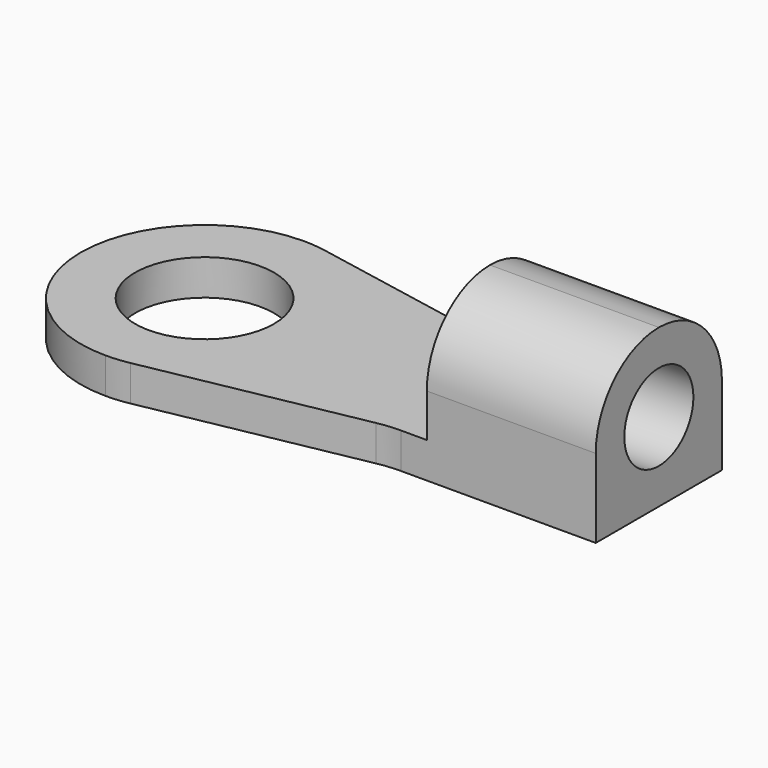
from build123d import *

# Parameters (mm, degrees)
F0_R     = 1.85
F1_DEPTH = 0.95
F2_W     = 4.5
F2_H     = 4.2
F3_DEPTH = 3.25
F4_R     = 2.09999
F5_R     = 1.15
F6_DEPTH = 25


# Not quite as in the source:
# - a fillet or chamfer is up to 0.001 mm smaller than in the source, because OpenCascade refuses the exact size


with BuildPart() as f1:
    # F0 (on Top) → F1 (new body)
    with BuildSketch(Plane.XY):
        with BuildLine():
            Line((10.9, 1.2), (15.4, 1.2))
            Line((15.4, 1.2), (15.4, 5.4))
            Line((15.4, 5.4), (10.9, 5.4))
            Line((10.9, 5.4), (10.2120730928, 5.4))
            ThreePointArc((10.2120730928, 5.4), (9.9013861494, 5.4146577616), (9.5934591909, 5.4585008344))
            Line((9.5934591909, 5.4585008344), (3.9186139019, 6.5414991656))
            ThreePointArc((3.9186139019, 6.5414991656), (3.6106869434, 6.5853422384), (3.3, 6.6))
            ThreePointArc((3.3, 6.6), (0.9665476221, 5.6334523779), (0, 3.3))
            ThreePointArc((0, 3.3), (0.9665476221, 0.9665476221), (3.3, 0))
            ThreePointArc((3.3, 0), (3.6106869434, 0.0146577616), (3.9186139019, 0.0585008344))
            Line((3.9186139019, 0.0585008344), (9.5934591909, 1.1414991656))
            ThreePointArc((9.5934591909, 1.1414991656), (9.9013861494, 1.1853422384), (10.2120730928, 1.2))
            Line((10.2120730928, 1.2), (10.9, 1.2))
        make_face()
        with Locations((3.3, 3.3)):
            Circle(F0_R, mode=Mode.SUBTRACT)
    extrude(amount=F1_DEPTH)

    # F2 (on face) → F3 (join)
    with BuildSketch(Plane.XY.offset(0.95)):
        with Locations((13.15, 3.3)):
            Rectangle(F2_W, F2_H)
    extrude(amount=F3_DEPTH)

    # F4 (radius 2.1 in the source; OpenCascade refuses exactly that, so slightly less here)
    f4_edges = [f1.edges().sort_by_distance(p)[0] for p in [
        (13.15, 5.4, 4.2),
        (13.15, 1.2, 4.2),
    ]]
    fillet(f4_edges, radius=F4_R)

    # F5 (on face) → F6 (cut)
    with BuildSketch(Plane.YZ.offset(15.4)):
        with Locations((3.3, 2.1)):
            Circle(F5_R)
    extrude(amount=-F6_DEPTH, mode=Mode.SUBTRACT)


solid = f1.part
